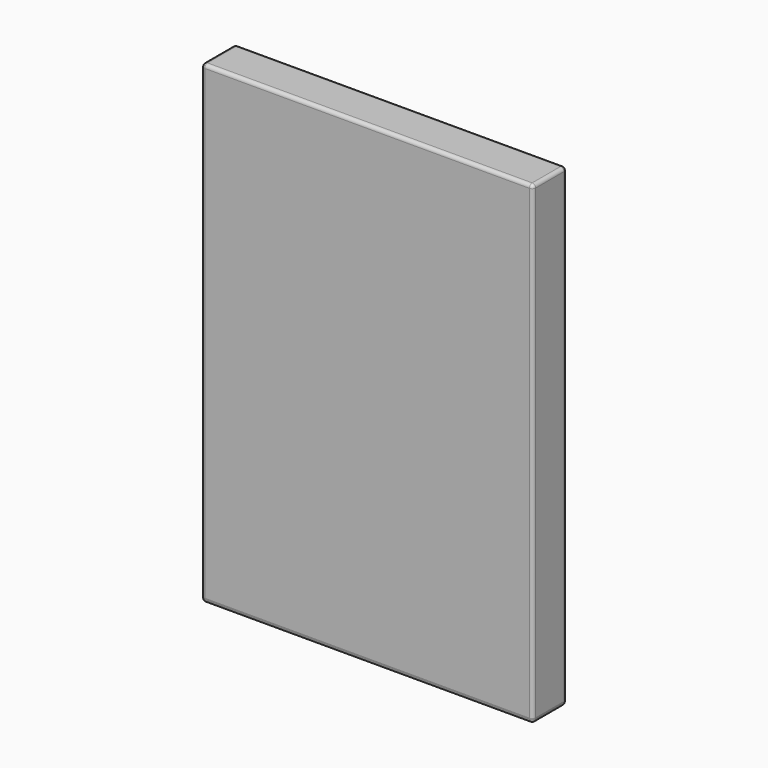
from build123d import *

# Parameters (mm, degrees)
F0_W          = 226.06
F0_H          = 325.12
F1_DEPTH      = 12.192
F2_W          = 245.11
F2_H          = 31.242
F2_W_2        = 238.76
F2_H_2        = 24.892
F3_DEPTH      = 337.82
F3_DEPTH_BACK = 6.35
F4_W          = 245.11
F4_H          = 31.242
F5_DEPTH      = 3.175
F6_W          = 245.11
F6_H          = 31.242
F7_DEPTH      = 3.175
F8_W          = 238.252
F8_H          = 24.384
F8_W_2        = 231.902
F8_H_2        = 18.034
F9_DEPTH      = 6.35
F10_R         = 2.54
F11_R         = 2.54
F11_2_R       = 2.54
F12_R         = 2.54
F12_2_R       = 2.54


# Not quite as in the source:
# - two fillets or chamfers of one size are made in one step


with BuildPart() as f1:
    # F0 (on Front) → F1 (new body)
    with BuildSketch(Plane.XZ):
        with Locations((113.03, 162.56)):
            Rectangle(F0_W, F0_H)
    extrude(amount=F1_DEPTH)


with BuildPart() as f3:
    # F2 (on face) → F3 (new body, two sides)
    with BuildSketch(Plane.XY.offset(325.12)) as f3_sk:
        with Locations((113.03, -6.096)):
            Rectangle(F2_W, F2_H)
        with Locations((113.03, -6.096)):
            Rectangle(F2_W_2, F2_H_2, mode=Mode.SUBTRACT)
    extrude(amount=-F3_DEPTH)
    extrude(f3_sk.sketch, amount=F3_DEPTH_BACK)

    # F4 (on face) → F5 (join)
    with BuildSketch(Plane.XY.offset(331.47)):
        with Locations((113.03, -6.096)):
            Rectangle(F4_W, F4_H)
    extrude(amount=F5_DEPTH)

    # F11
    f11_edges = [f3.edges().sort_by_distance(p)[0] for p in [
        (235.585, -21.717, 160.9725),
    ]]
    fillet(f11_edges, radius=F11_R)

    # F12
    f12_edges = [f3.edges().sort_by_distance(p)[0] for p in [
        (235.585, 9.525, 160.9725),
        (235.585, -4.826, 334.645),
        (234.841051, -20.973051, 334.645),
        (-9.525, 9.525, 160.9725),
        (113.03, 9.525, 334.645),
        (111.76, -21.717, 334.645),
        (-9.525, -6.096, 334.645),
        (-9.525, -21.717, 160.9725),
    ]]
    fillet(f12_edges, radius=F12_R)


with BuildPart() as f7:
    # F6 (on face) → F7 (new body)
    with BuildSketch(Plane(origin=(0, 0, -12.7), x_dir=(1, 0, 0), z_dir=(0, 0, -1))):
        with Locations((113.03, 6.096)):
            Rectangle(F6_W, F6_H)
    extrude(amount=F7_DEPTH)

    # F8 (on face) → F9 (join)
    with BuildSketch(Plane.XY.offset(-12.7)):
        with Locations((113.03, -6.096)):
            Rectangle(F8_W, F8_H)
        with Locations((113.03, -6.096)):
            Rectangle(F8_W_2, F8_H_2, mode=Mode.SUBTRACT)
    extrude(amount=F9_DEPTH)

    # F10
    f10_edges = [f7.edges().sort_by_distance(p)[0] for p in [
        (235.585, -6.096, -15.875),
    ]]
    fillet(f10_edges, radius=F10_R)

    # F11#2
    f11_2_edges = [f7.edges().sort_by_distance(p)[0] for p in [
        (111.76, 9.525, -15.875),
    ]]
    fillet(f11_2_edges, radius=F11_2_R)

    # F12#2
    f12_2_edges = [f7.edges().sort_by_distance(p)[0] for p in [
        (235.585, -21.717, -13.0175),
        (234.841051, -21.717, -15.131051),
        (111.76, -21.717, -15.875),
        (-9.525, -21.717, -14.2875),
        (-9.525, -7.366, -15.875),
        (-9.525, 9.525, -13.0175),
        (-9.525, 8.781051, -15.131051),
    ]]
    fillet(f12_2_edges, radius=F12_2_R)


solid = Compound([f1.part, f3.part, f7.part])
